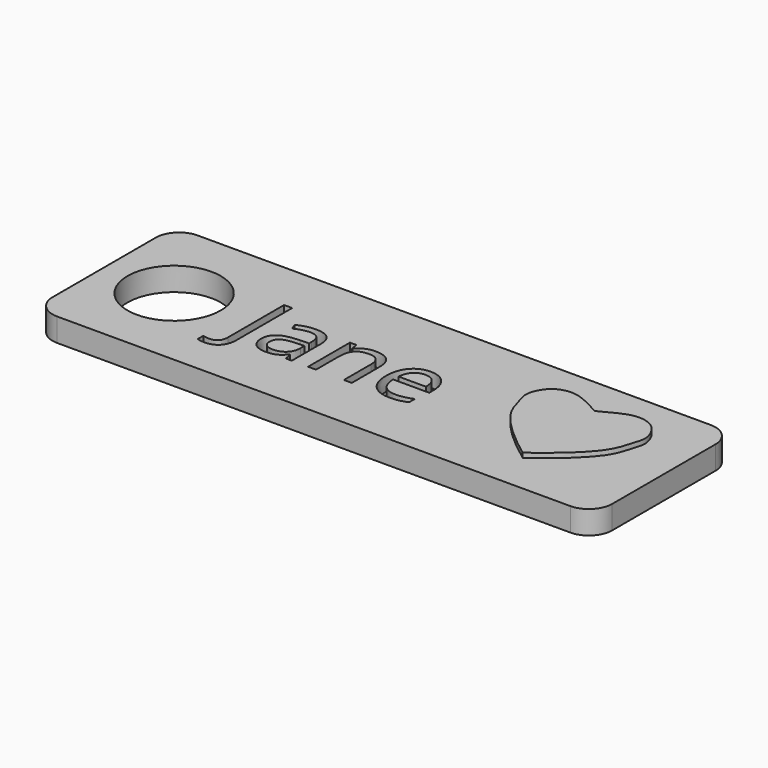
from build123d import *

# Parameters (mm, degrees)
F0_W         = 120
F0_H         = 37.6530177891
F0_R         = 10
F1_DEPTH     = 5
F2_R         = 5
F3_TEXT_SIZE = 20.9703963871
F4_DEPTH     = 3
F7_DEPTH     = 6


# Not quite as in the source:
# - Text() gives the source's letters only with a copy of the font that has no kerning and outlines rounded to 1/6400 em; it was checked with that copy


with BuildPart() as f1:
    # F0 (on Top) → F1 (new body)
    with BuildSketch(Plane.XY):
        Rectangle(F0_W, F0_H)
        with Locations((-45, 0)):
            Circle(F0_R, mode=Mode.SUBTRACT)
    extrude(amount=F1_DEPTH)

    # F2
    f2_edges = [f1.edges().sort_by_distance(p)[0] for p in [
        (60, 18.826509, 2.5),
        (-60, 18.826509, 2.5),
        (-60, -18.826509, 2.5),
        (60, -18.826509, 2.5),
    ]]
    fillet(f2_edges, radius=F2_R)

    # F3 (on face) → F4 (cut)
    with BuildSketch(Plane.XY.offset(5)):
        with Locations((-29.9013182521, -6.8092113361)):
            Text('Jane', F3_TEXT_SIZE, font='Open Sans', text_align=(TextAlign.LEFT, TextAlign.BOTTOM))
    extrude(amount=-F4_DEPTH, mode=Mode.SUBTRACT)

    # F6 (on Top) → F7 (join)
    with BuildSketch(Plane.XY):
        with BuildLine():
            add(Edge.make_bspline(
                [(37.8947407007, 9.1561628506), (39.7079815693, 10.1322071832), (42.8020396326, 11.797699005), (45.729148546, 12.1456175543), (49.0567279025, 11.1487902134), (51.1473677312, 7.0340855028), (50.0110767523, 4.0410866304), (48.9773979812, -0.400333582), (43.1661068035, -6.2224068524), (39.596914473, -8.9031274091), (37.8947407007, -10.1815825328)],
                knots=[0, 0, 0, 0, 0.1384934947, 0.2363210104, 0.3407802777, 0.4593986422, 0.560619941, 0.6829605476, 0.8488015801, 1, 1, 1, 1], degree=3))
            add(Edge.make_bspline(
                [(37.8947407007, 9.1561628506), (36.0814998321, 10.1322071832), (32.9874417689, 11.797699005), (30.0603328554, 12.1456175543), (26.7327534989, 11.1487902134), (24.6421136702, 7.0340855028), (25.7784046492, 4.0410866304), (26.8120834203, -0.400333582), (32.6233745979, -6.2224068524), (36.1925669284, -8.9031274091), (37.8947407007, -10.1815825328)],
                knots=[0, 0, 0, 0, 0.1384934947, 0.2363210104, 0.3407802777, 0.4593986422, 0.560619941, 0.6829605476, 0.8488015801, 1, 1, 1, 1], degree=3))
        make_face()
    extrude(amount=F7_DEPTH)


solid = f1.part
